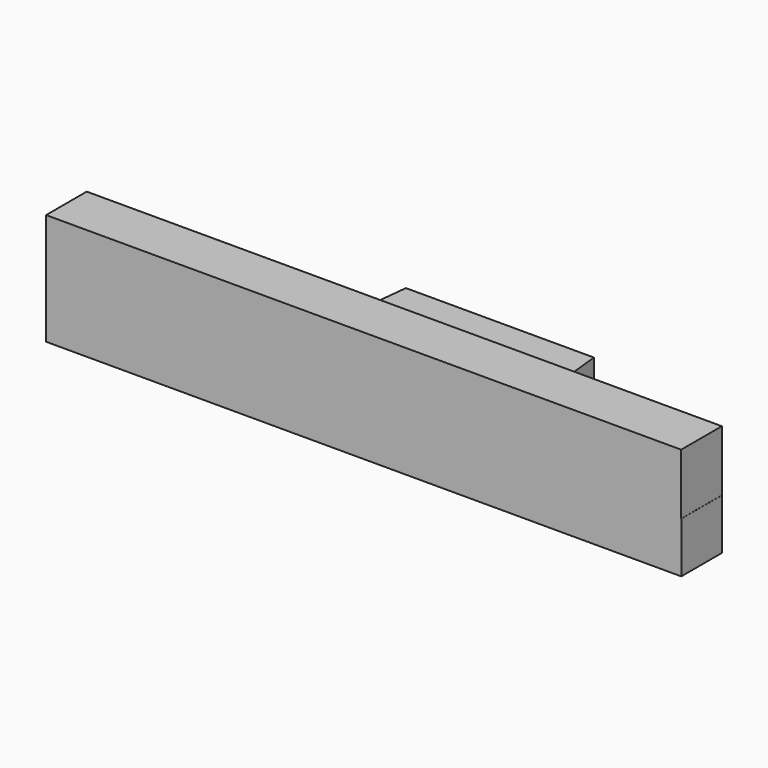
from build123d import *

# Parameters (mm, degrees)
F1_DEPTH      = 200
F2_W          = 200
F2_H          = 240
F3_DEPTH      = 2294
F3_DEPTH_BACK = 206
F4_T          = -2.5


with BuildPart() as f1:
    # F0 (on Top) → F1 (new body)
    with BuildSketch(Plane.XY):
        Polygon((-205.6466794014, 200), (-205.6466794014, 0), (2294.3533205986, 0), (2294.3533205986, 200), (1464.3533205986, 200), (1044.3533205986, 200), (624.3533205986, 200), align=None)
        Polygon((674.3533205986, 670), (624.3533205986, 200), (1044.3533205986, 200), (1044.3533205986, 670), align=None)
        Polygon((1044.3533205986, 200), (1464.3533205986, 200), (1414.3533205986, 670), (1044.3533205986, 670), align=None)
    extrude(amount=F1_DEPTH)

    # F2 (on Right) → F3 (join, two sides)
    with BuildSketch(Plane.YZ) as f3_sk:
        with Locations((100, 319.0685760975)):
            Rectangle(F2_W, F2_H)
    extrude(amount=F3_DEPTH)
    extrude(f3_sk.sketch, amount=-F3_DEPTH_BACK)

    # F4
    f4_openings = [f1.faces().sort_by_distance(p)[0] for p in [
        (1044.353321, 670, 100),
    ]]
    offset(amount=F4_T, openings=f4_openings, kind=Kind.INTERSECTION)


solid = f1.part
